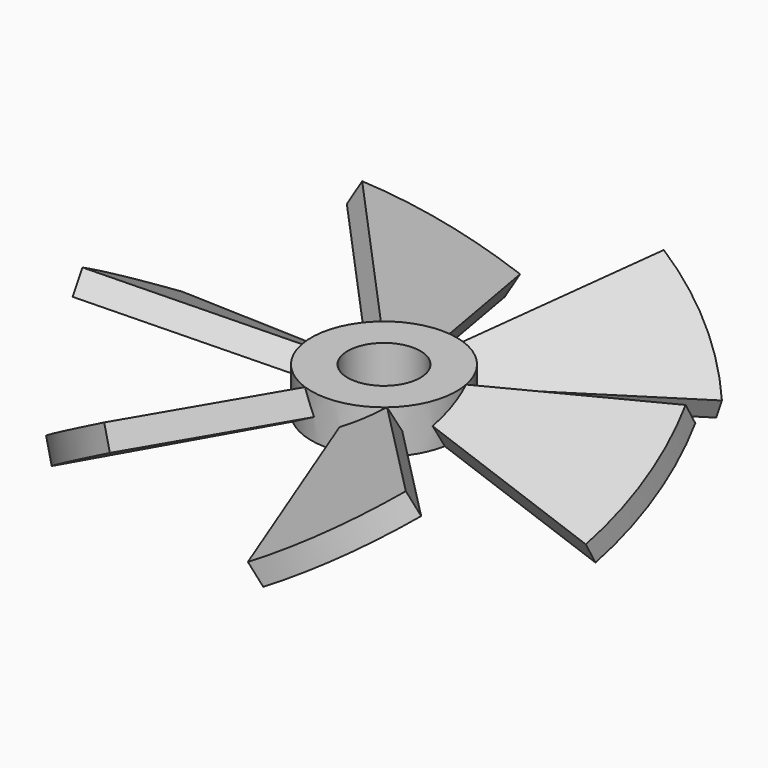
from build123d import *

# Parameters (mm, degrees)
F3_DEPTH      = 5
F3_DEPTH_BACK = 5
F5_COUNT      = 6
F6_R          = 30
F7_DEPTH      = 20
F7_DEPTH_BACK = 20
F9_R          = 30
F10_DEPTH     = 25
F12_R         = 30
F13_DEPTH     = 25
F14_R         = 15
F15_DEPTH     = 25


with BuildPart() as f3:
    # F2 (on face) → F3 (new body, two sides)
    with BuildSketch(Plane(origin=(0, 0, 0), x_dir=(1, 0, 0), z_dir=(0, 0.5, -0.8660254038))) as f3_sk:
        with BuildLine():
            Line((0, -1.3531434218), (105.9060541663, -29.7305851092))
            ThreePointArc((105.9060541663, -29.7305851092), (110, 0), (105.9060541663, 29.7305851092))
            Line((105.9060541663, 29.7305851092), (-5.05, 0))
            Line((-5.05, 0), (0, 0))
            Line((0, 0), (0, -1.3531434218))
        make_face()
    extrude(amount=F3_DEPTH)
    extrude(f3_sk.sketch, amount=-F3_DEPTH_BACK)

    # F5: F3 ×6 about axis
    f5_axis = Axis((0, 0, 14.0805), (0, 0, 1))


with BuildPart() as f3_1:
    add(f3.part)
    for i in range(1, F5_COUNT):
        add(f3.part.rotate(f5_axis, i * 360 / F5_COUNT))

    # F6 (on Top) → F7 (join, two sides)
    with BuildSketch(Plane.XY) as f7_sk:
        Circle(F6_R)
    extrude(amount=F7_DEPTH)
    extrude(f7_sk.sketch, amount=-F7_DEPTH_BACK)

    # F9 (on plane+point) → F10 (cut)
    with BuildSketch(Plane.XY.offset(8.9574447446)):
        Circle(F9_R)
    extrude(amount=F10_DEPTH, mode=Mode.SUBTRACT)

    # F12 (on plane+point) → F13 (cut)
    with BuildSketch(Plane.XY.offset(-8.9574447446)):
        Circle(F12_R)
    extrude(amount=-F13_DEPTH, mode=Mode.SUBTRACT)

    # F14 (on face) → F15 (cut)
    with BuildSketch(Plane(origin=(0, 0, -8.9574447446), x_dir=(1, 0, 0), z_dir=(0, 0, -1))):
        Circle(F14_R)
    extrude(amount=-F15_DEPTH, mode=Mode.SUBTRACT)


solid = f3_1.part
